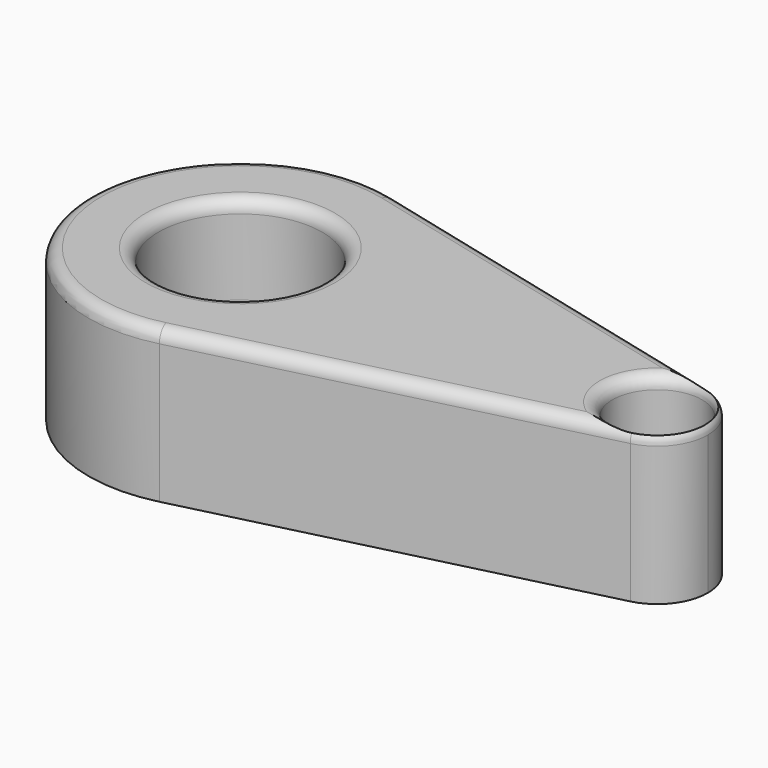
from build123d import *

# Parameters (mm, degrees)
F1_DEPTH     = 76.2
F2_R         = 22.557617544
F2_R_2       = 41.140256543
F3_DEPTH     = 50.8
F4_T5_DEPTH  = 203.2
F4_T7_DEPTH  = 203.2
F4_T10_ANGLE = 151.9275130641
F4_T12_ANGLE = 208.0724869359
F5_T         = -2.54


# Not quite as in the source:
# - a fillet or chamfer that OpenCascade refuses, or shapes differently, is made with other operations: its cross-section is extruded or revolved along the edge and cut away or added


with BuildPart() as f1:
    # F0 (on Top) → F1 (new body)
    with BuildSketch(Plane.XY):
        with BuildLine():
            ThreePointArc((18.4812146278, 73.9248585111), (60.0612543768, 46.8944103565), (76.2, 0))
            ThreePointArc((76.2, 0), (60.0612543768, -46.8944103565), (18.4812146278, -73.9248585111))
            Line((18.4812146278, -73.9248585111), (215.6141706573, -24.6416195037))
            ThreePointArc((215.6141706573, -24.6416195037), (184.0537657814, 0), (215.6141706573, 24.6416195037))
            Line((215.6141706573, 24.6416195037), (18.4812146278, 73.9248585111))
        make_face()
        with BuildLine():
            ThreePointArc((18.4812146278, -73.9248585111), (60.0612543768, -46.8944103565), (76.2, 0))
            ThreePointArc((76.2, 0), (60.0612543768, 46.8944103565), (18.4812146278, 73.9248585111))
            ThreePointArc((18.4812146278, 73.9248585111), (-76.2, 0), (18.4812146278, -73.9248585111))
        make_face()
        with BuildLine():
            ThreePointArc((234.8537657814, 0), (229.474183907, 15.6314701188), (215.6141706573, 24.6416195037))
            ThreePointArc((215.6141706573, 24.6416195037), (184.0537657814, 0), (215.6141706573, -24.6416195037))
            ThreePointArc((215.6141706573, -24.6416195037), (229.474183907, -15.6314701188), (234.8537657814, 0))
        make_face()
    extrude(amount=F1_DEPTH)

    # F2 (on face) → F3 (cut)
    with BuildSketch(Plane.XY.offset(76.2)):
        with Locations((209.4537657814, 0)):
            Circle(F2_R)
        Circle(F2_R_2)
    extrude(amount=-F3_DEPTH, mode=Mode.SUBTRACT)

    # F4: fillet of radius 6.35 on 8 edges, made by hand

    # F4_s1 → F4_t2 (revolve)
    with BuildSketch(Plane.XZ):
        with BuildLine():
            ThreePointArc((41.140256543, 31.75), (39.2803846036, 27.2598719395), (34.790256543, 25.4))
            Line((34.790256543, 25.4), (41.140256543, 25.4))
            Line((41.140256543, 25.4), (41.140256543, 31.75))
        make_face()
    revolve(axis=Axis((0, 0, 25.4), (0, 0, 1)))

    # F4_s3 → F4_t4 (revolve)
    with BuildSketch(Plane.XZ):
        with BuildLine():
            ThreePointArc((232.0113833254, 31.75), (230.151511386, 27.2598719395), (225.6613833254, 25.4))
            Line((225.6613833254, 25.4), (232.0113833254, 25.4))
            Line((232.0113833254, 25.4), (232.0113833254, 31.75))
        make_face()
    revolve(axis=Axis((209.4537657814, 0, 25.4), (0, 0, 1)))

    # F4_s6 → F4_t5 (cut)
    with BuildSketch(Plane(origin=(0, 0, 0), x_dir=(0, 0, 1), z_dir=(0.9701425001, 0.242535625, 0))):
        with BuildLine():
            ThreePointArc((76.2, 69.85), (74.3401280605, 74.3401280605), (69.85, 76.2))
            Line((69.85, 76.2), (76.2, 76.2))
            Line((76.2, 76.2), (76.2, 69.85))
        make_face()
    extrude(amount=F4_T5_DEPTH, mode=Mode.SUBTRACT)

    # F4_s8 → F4_t7 (cut)
    with BuildSketch(Plane(origin=(197.1329560295, -49.2832390074, 0), x_dir=(0, 0, 1), z_dir=(-0.9701425001, 0.242535625, 0))):
        with BuildLine():
            ThreePointArc((69.85, 76.2), (74.3401280605, 74.3401280605), (76.2, 69.85))
            Line((76.2, 69.85), (76.2, 76.2))
            Line((76.2, 76.2), (69.85, 76.2))
        make_face()
    extrude(amount=F4_T7_DEPTH, mode=Mode.SUBTRACT)

    # F4_s9 → F4_t10 (revolve, cut)
    with BuildSketch(Plane(origin=(197.1329560295, 49.2832390074, 0), x_dir=(0, 0, 1), z_dir=(-0.9701425001, -0.242535625, 0))):
        with BuildLine():
            ThreePointArc((69.85, -76.2), (74.3401280605, -74.3401280605), (76.2, -69.85))
            Line((76.2, -69.85), (76.2, -76.2))
            Line((76.2, -76.2), (69.85, -76.2))
        make_face()
    revolve(axis=Axis((209.4537657814, 0, 76.2), (0, 0, 1)), revolution_arc=F4_T10_ANGLE, mode=Mode.SUBTRACT)

    # F4_s11 → F4_t12 (revolve, cut)
    with BuildSketch(Plane(origin=(0, 0, 0), x_dir=(0, 0, 1), z_dir=(0.9701425001, -0.242535625, 0))):
        with BuildLine():
            ThreePointArc((69.85, -76.2), (74.3401280605, -74.3401280605), (76.2, -69.85))
            Line((76.2, -69.85), (76.2, -76.2))
            Line((76.2, -76.2), (69.85, -76.2))
        make_face()
    revolve(axis=Axis((0, 0, 76.2), (0, 0, 1)), revolution_arc=F4_T12_ANGLE, mode=Mode.SUBTRACT)

    # F4_s13 → F4_t14 (revolve, cut)
    with BuildSketch(Plane.XZ):
        with BuildLine():
            ThreePointArc((238.3613833254, 76.2), (233.8712552649, 74.3401280605), (232.0113833254, 69.85))
            Line((232.0113833254, 69.85), (232.0113833254, 76.2))
            Line((232.0113833254, 76.2), (238.3613833254, 76.2))
        make_face()
    revolve(axis=Axis((209.4537657814, 0, 76.2), (0, 0, 1)), mode=Mode.SUBTRACT)

    # F4_s15 → F4_t16 (revolve, cut)
    with BuildSketch(Plane.XZ):
        with BuildLine():
            ThreePointArc((47.490256543, 76.2), (43.0001284825, 74.3401280605), (41.140256543, 69.85))
            Line((41.140256543, 69.85), (41.140256543, 76.2))
            Line((41.140256543, 76.2), (47.490256543, 76.2))
        make_face()
    revolve(axis=Axis((0, 0, 76.2), (0, 0, 1)), mode=Mode.SUBTRACT)

    # F5
    f5_openings = [f1.faces().sort_by_distance(p)[0] for p in [
        (57.51924, 0, 0),
    ]]
    offset(amount=F5_T, openings=f5_openings)


solid = f1.part
